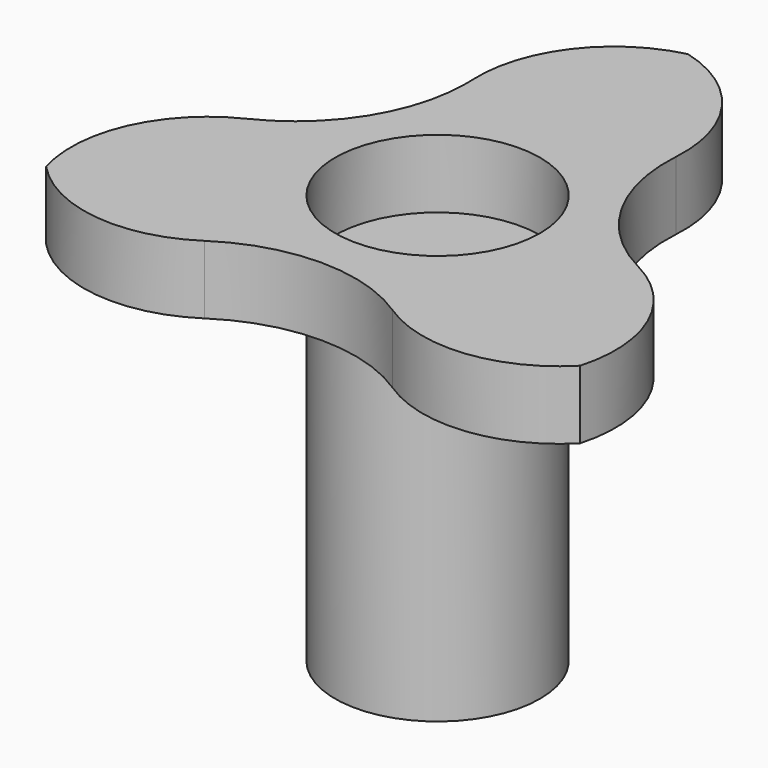
from build123d import *

# Parameters (mm, degrees)
F0_R        = 3.81
F1_DEPTH    = 12.7
F2_R        = 3.81
F3_DEPTH    = 2.54
F4_T1_DEPTH = 42.0384776465


# Not quite as in the source:
# - a fillet or chamfer that OpenCascade refuses, or shapes differently, is made with other operations: its cross-section is extruded or revolved along the edge and cut away or added


with BuildPart() as f1:
    # F0 (on Top) → F1 (new body)
    with BuildSketch(Plane.XY):
        Circle(F0_R)
    extrude(amount=F1_DEPTH)


with BuildPart() as f3:
    # F2 (on face) → F3 (new body)
    with BuildSketch(Plane.XY.offset(12.7)):
        with BuildLine():
            ThreePointArc((11.7509897523, -0.35949854), (4.7016682053, 2.6691615996), (5.7140252702, 10.274478798))
            ThreePointArc((5.7140252702, 10.274478798), (0.1269192039, 11.7558024343), (-5.4908664559, 10.3954502029))
            ThreePointArc((-5.4908664559, 10.3954502029), (-4.1984383287, 8.3771195895), (-3.7461525862, 6.0235124566))
            ThreePointArc((-3.7461525862, 6.0235124566), (-6.2372414103, 0.980566439), (-11.7560122827, -0.1057098259))
            ThreePointArc((-11.7560122827, -0.1057098259), (-10.2232663206, -5.8051550451), (-6.1140496846, -10.041583332))
            ThreePointArc((-6.1140496846, -10.041583332), (0, -5.4064875434), (6.1140496846, -10.041583332))
            ThreePointArc((6.1140496846, -10.041583332), (10.16, -5.9151837975), (11.7509897523, -0.35949854))
        make_face()
        Circle(F2_R, mode=Mode.SUBTRACT)
    extrude(amount=F3_DEPTH)

    # F4: fillet of radius 5.08 on 6 edges, made by hand

    # F4_s2 → F4_t1 (cut)
    with BuildSketch(Plane.XY.offset(-7.0492388233)):
        with BuildLine():
            ThreePointArc((7.3426084647, 0.1454248286), (10.0242781389, -3.4122038252), (8.8706351528, -7.7153633319))
            ThreePointArc((8.8706351528, -7.7153633319), (10.9471475801, -4.2866022929), (11.7509897523, -0.35949854))
            ThreePointArc((11.7509897523, -0.35949854), (9.5012608724, -0.5046217571), (7.3426084647, 0.1454248286))
        make_face()
        with BuildLine():
            ThreePointArc((3.888167348, 6.230345265), (2.2077692466, 10.3564010208), (-2.0785006989, 11.5712935406))
            ThreePointArc((-2.0785006989, 11.5712935406), (1.9299460735, 11.5969956244), (5.7140252702, 10.274478798))
            ThreePointArc((5.7140252702, 10.274478798), (4.4363623338, 8.4170832554), (3.888167348, 6.230345265))
        make_face()
        with BuildLine():
            ThreePointArc((-3.7527473325, 6.3128388943), (-1.9836590084, 10.4016529498), (2.3278414748, 11.5237213359))
            ThreePointArc((2.3278414748, 11.5237213359), (-1.6791160458, 11.6359601522), (-5.4908664559, 10.3954502029))
            ThreePointArc((-5.4908664559, 10.3954502029), (-4.2536026695, 8.5109027497), (-3.7527473325, 6.3128388943))
        make_face()
        with BuildLine():
            ThreePointArc((-9.0351428515, -7.522047129), (-10.0956113335, -3.1949834043), (-7.337757218, 0.3039185031))
            ThreePointArc((-7.337757218, 0.3039185031), (-9.5099410225, -0.299371063), (-11.7560122827, -0.1057098259))
            ThreePointArc((-11.7560122827, -0.1057098259), (-11.0371440012, -4.0492532221), (-9.0351428515, -7.522047129))
        make_face()
        with BuildLine():
            ThreePointArc((-3.4985504193, -6.4571814602), (-7.9163168625, -7.0328667329), (-11.088943922, -3.9051660725))
            ThreePointArc((-11.088943922, -3.9051660725), (-9.1323409623, -7.4037387789), (-6.1140496846, -10.041583332))
            ThreePointArc((-6.1140496846, -10.041583332), (-5.1295715595, -8.0134946746), (-3.4985504193, -6.4571814602))
        make_face()
        with BuildLine():
            ThreePointArc((3.4985504193, -6.4571814602), (7.9163168625, -7.0328667329), (11.088943922, -3.9051660725))
            ThreePointArc((11.088943922, -3.9051660725), (9.1323409623, -7.4037387789), (6.1140496846, -10.041583332))
            ThreePointArc((6.1140496846, -10.041583332), (5.1295715595, -8.0134946746), (3.4985504193, -6.4571814602))
        make_face()
    extrude(amount=F4_T1_DEPTH, mode=Mode.SUBTRACT)


solid = Compound([f1.part, f3.part])
